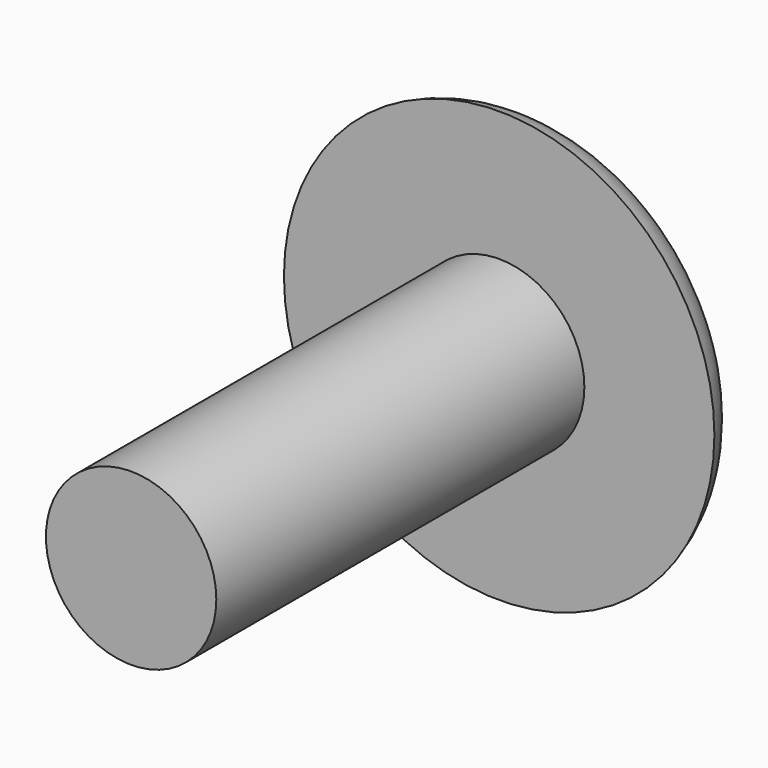
from build123d import *

# Parameters (mm, degrees)
F0_R     = 2.5
F1_DEPTH = 15
F0_R_2   = 6.3158003242
F2_DEPTH = 1.5


# Not quite as in the source:
# - a fillet or chamfer that OpenCascade refuses, or shapes differently, is made with other operations: its cross-section is extruded or revolved along the edge and cut away or added


with BuildPart() as f1:
    # F0 (on Front) → F1 (new body)
    with BuildSketch(Plane.XZ):
        Circle(F0_R)
    extrude(amount=F1_DEPTH)

    # F0 (on Front) → F2 (join)
    with BuildSketch(Plane.XZ):
        Circle(F0_R_2)
        Circle(F0_R, mode=Mode.SUBTRACT)
    extrude(amount=F2_DEPTH)

    # F3: fillet of radius 2 on 1 edges, made by hand

    # F3_s1 → F3_t2 (revolve, cut)
    with BuildSketch(Plane.XY):
        with BuildLine():
            ThreePointArc((6.3158003242, -1.5), (5.6040535225, -0.4188611699), (4.3793086511, 0))
            Line((4.3793086511, 0), (6.3158003242, 0))
            Line((6.3158003242, 0), (6.3158003242, -1.5))
        make_face()
    revolve(axis=Axis((0, 0, 0), (0, -1, 0)), mode=Mode.SUBTRACT)


solid = f1.part
